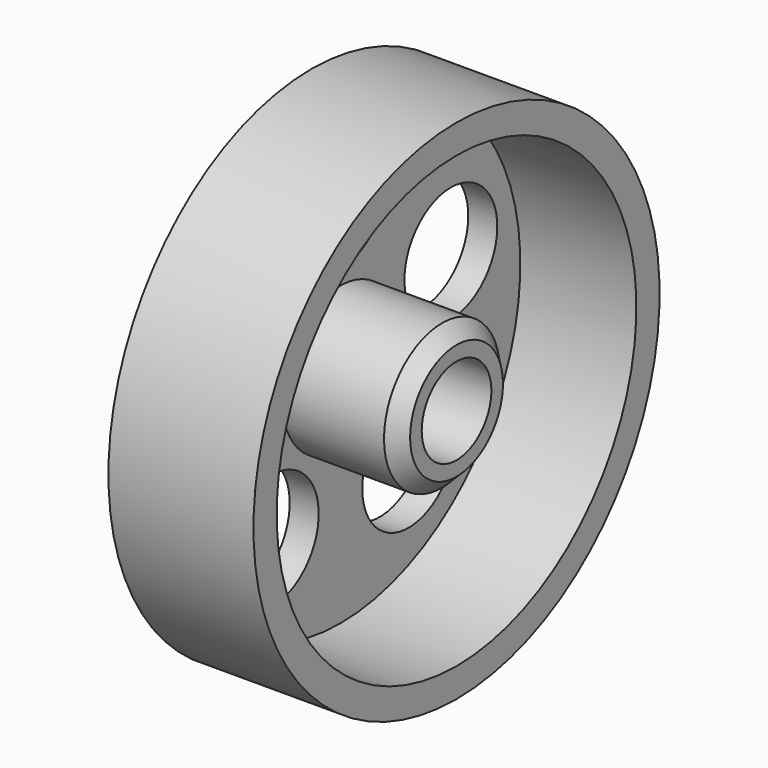
from build123d import *

# Parameters (mm, degrees)
F0_W            = 10
F0_H            = 17.5
F3_D            = 6
F4_T            = -2
F6_D            = 8
F6_COPIES_COUNT = 5
F7_SIZE         = 1


# Not quite as in the source:
# - a pattern or mirror of a feature is missing from the dataset's text; its kind, count and spacing are read off the source's solid


with BuildPart() as f1:
    # F0 (on Front) → F1 (revolve)
    with BuildSketch(Plane.XZ):
        with Locations((5, 8.75)):
            Rectangle(F0_W, F0_H)
    revolve(axis=Axis((5, 0, 0), (1, 0, 0)))

    # F3 (through all)
    with Locations(Plane(origin=(0, 0, 0), x_dir=(0, 1, 0), z_dir=(-1, 0, 0))):
        with Locations((0, 0)):
            Hole(F3_D / 2)

    # F4
    f4_openings = [f1.faces().sort_by_distance(p)[0] for p in [
        (10, 0, -17.005025),
    ]]
    offset(amount=F4_T, openings=f4_openings)

    # F6 (through all)
    with Locations(Plane(origin=(0, 0, 0), x_dir=(0, -1, 0), z_dir=(-1, 0, 0))):
        with Locations((0, 10)):
            f6 = Hole(F6_D / 2)

    # F6_copies: F6 ×5 about axis
    f6_copies_axis = Axis((0, 0, 0), (1, 0, 0))
    for i in range(1, F6_COPIES_COUNT):
        add(f6.rotate(f6_copies_axis, i * 360 / F6_COPIES_COUNT), mode=Mode.SUBTRACT)

    # F7
    f7_edges = [f1.edges().sort_by_distance(p)[0] for p in [
        (10, -5, 0),
    ]]
    chamfer(f7_edges, length=F7_SIZE)


solid = f1.part
